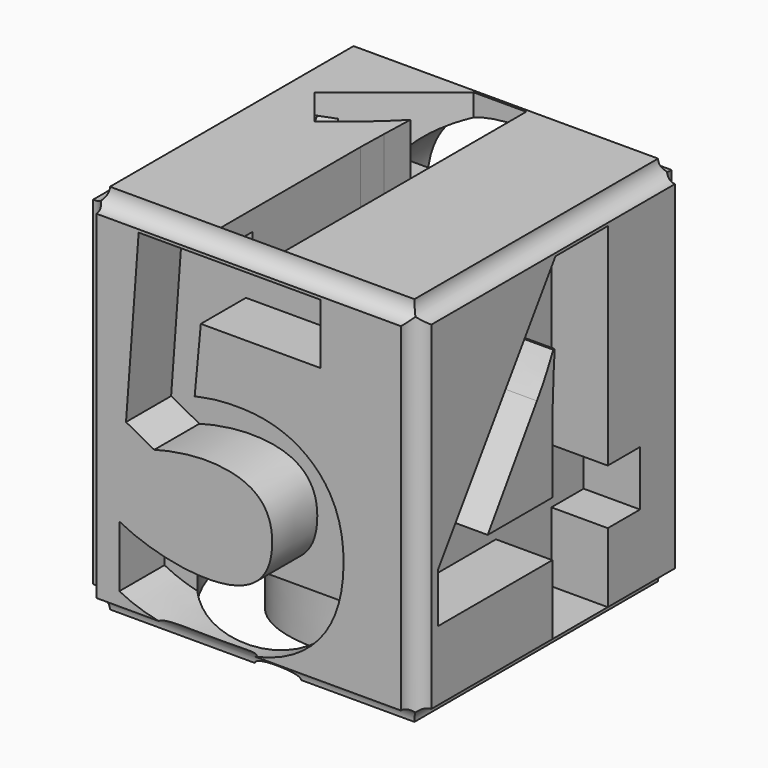
from build123d import *

# Parameters (mm, degrees)
F1_DEPTH      = 33
F2_R          = 1.5
F3_DEPTH      = 30.001
F4_R          = 1.5
F5_DEPTH      = 30.001
F6_R          = 1.5
F7_DEPTH      = 30.001
F8_R          = 1.5
F9_DEPTH      = 30.001
F10_R         = 1.5
F11_DEPTH     = 30.001
F12_R         = 1.5
F13_DEPTH     = 30.001
F14_TEXT_SIZE = 37.5
F15_DEPTH     = 5
F16_TEXT_SIZE = 37.5
F17_DEPTH     = 5
F18_TEXT_SIZE = 41.6666666667
F19_DEPTH     = 5
F20_TEXT_SIZE = 41.6666666667
F21_DEPTH     = 5
F22_TEXT_SIZE = 41.6666666667
F23_DEPTH     = 5
F24_TEXT_SIZE = 41.6666666667
F25_DEPTH     = 5


# Not quite as in the source:
# - Text() gives the source's letters only with a copy of the font that has no kerning and outlines rounded to 1/6400 em; it was checked with that copy


with BuildPart() as f1:
    # F0 (on Top) → F1 (new body)
    with BuildSketch(Plane.XY):
        with BuildLine():
            ThreePointArc((0, 1.5), (1.0606601718, 1.0606601718), (1.5, 0))
            Line((1.5, 0), (28.5, 0))
            ThreePointArc((28.5, 0), (28.9393398282, 1.0606601718), (30, 1.5))
            Line((30, 1.5), (30, 28.5))
            ThreePointArc((30, 28.5), (28.9393398282, 28.9393398282), (28.5, 30))
            Line((28.5, 30), (1.5, 30))
            ThreePointArc((1.5, 30), (1.0606601718, 28.9393398282), (0, 28.5))
            Line((0, 28.5), (0, 1.5))
        make_face()
    extrude(amount=F1_DEPTH)

    # F2 (on Right) → F3 (cut, through all)
    with BuildSketch(Plane.YZ):
        with Locations((0, 33)):
            Circle(F2_R)
    extrude(amount=F3_DEPTH, mode=Mode.SUBTRACT)

    # F4 (on Front) → F5 (cut, through all)
    with BuildSketch(Plane.XZ):
        with Locations((30, 33)):
            Circle(F4_R)
    extrude(amount=-F5_DEPTH, mode=Mode.SUBTRACT)

    # F6 (on Right) → F7 (cut, through all)
    with BuildSketch(Plane.YZ):
        Circle(F6_R)
        with Locations((30, 0)):
            Circle(F6_R)
    extrude(amount=F7_DEPTH, mode=Mode.SUBTRACT)

    # F8 (on Right) → F9 (cut, through all)
    with BuildSketch(Plane.YZ):
        with Locations((30, 33)):
            Circle(F8_R)
    extrude(amount=F9_DEPTH, mode=Mode.SUBTRACT)

    # F10 (on Front) → F11 (cut, through all)
    with BuildSketch(Plane.XZ):
        with Locations((30, 0)):
            Circle(F10_R)
        Circle(F10_R)
    extrude(amount=-F11_DEPTH, mode=Mode.SUBTRACT)

    # F12 (on Front) → F13 (cut, through all)
    with BuildSketch(Plane.XZ):
        with Locations((0, 33)):
            Circle(F12_R)
    extrude(amount=-F13_DEPTH, mode=Mode.SUBTRACT)

    # F14 (on face) → F15 (cut)
    with BuildSketch(Plane.XY.offset(33)):
        with Locations((1.5, 1.5)):
            Text('1', F14_TEXT_SIZE, font='Open Sans', font_style=FontStyle.BOLD, text_align=(TextAlign.LEFT, TextAlign.BOTTOM))
    extrude(amount=-F15_DEPTH, mode=Mode.SUBTRACT)

    # F16 (on face) → F17 (cut)
    with BuildSketch(Plane(origin=(0, 0, 0), x_dir=(1, 0, 0), z_dir=(0, 0, -1))):
        with Locations((1.5, -28.5)):
            Text('6', F16_TEXT_SIZE, font='Open Sans', font_style=FontStyle.BOLD, text_align=(TextAlign.LEFT, TextAlign.BOTTOM))
    extrude(amount=-F17_DEPTH, mode=Mode.SUBTRACT)

    # F18 (on face) → F19 (cut)
    with BuildSketch(Plane.YZ.offset(30)):
        with Locations((1.5, 1.5)):
            Text('4', F18_TEXT_SIZE, font='Open Sans', font_style=FontStyle.BOLD, text_align=(TextAlign.LEFT, TextAlign.BOTTOM))
    extrude(amount=-F19_DEPTH, mode=Mode.SUBTRACT)

    # F20 (on face) → F21 (cut)
    with BuildSketch(Plane(origin=(0, 0, 0), x_dir=(0, -1, 0), z_dir=(-1, 0, 0))):
        with Locations((-28.5, 1.5)):
            Text('3', F20_TEXT_SIZE, font='Open Sans', font_style=FontStyle.BOLD, text_align=(TextAlign.LEFT, TextAlign.BOTTOM))
    extrude(amount=-F21_DEPTH, mode=Mode.SUBTRACT)

    # F22 (on face) → F23 (cut)
    with BuildSketch(Plane.XZ):
        with Locations((1.5, 1.5)):
            Text('5', F22_TEXT_SIZE, font='Open Sans', font_style=FontStyle.BOLD, text_align=(TextAlign.LEFT, TextAlign.BOTTOM))
    extrude(amount=-F23_DEPTH, mode=Mode.SUBTRACT)

    # F24 (on face) → F25 (cut)
    with BuildSketch(Plane(origin=(0, 30, 0), x_dir=(-1, 0, 0), z_dir=(0, 1, 0))):
        with Locations((-28.5, 1.5)):
            Text('2', F24_TEXT_SIZE, font='Open Sans', font_style=FontStyle.BOLD, text_align=(TextAlign.LEFT, TextAlign.BOTTOM))
    extrude(amount=-F25_DEPTH, mode=Mode.SUBTRACT)


solid = f1.part
